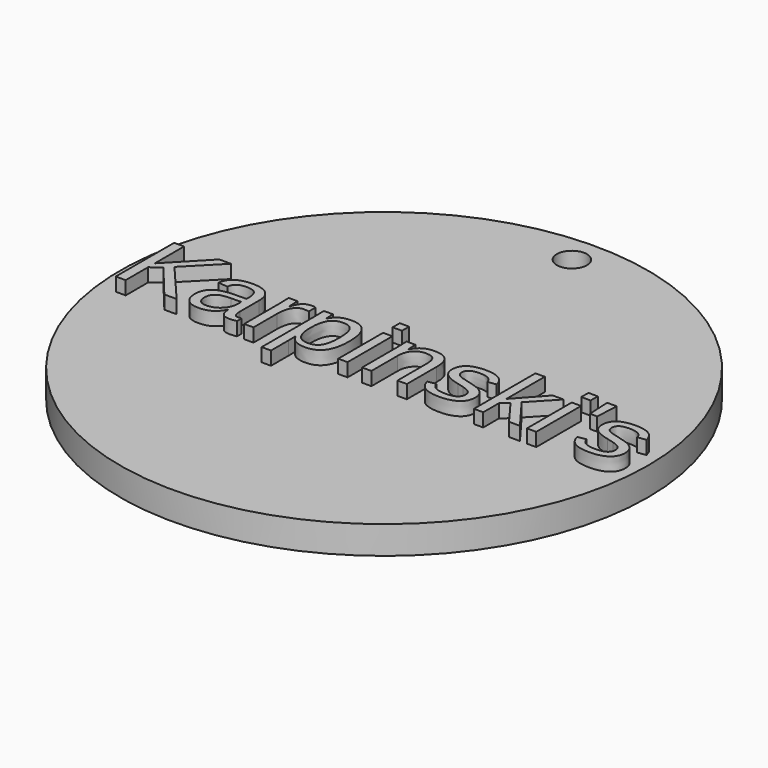
from build123d import *

# Parameters (mm, degrees)
F0_R         = 59.8348431243
F1_DEPTH     = 6.35
F2_TEXT_SIZE = 24.0505336827
F3_DEPTH     = 3.048
F4_R         = 3.4124645747
F5_DEPTH     = 25.4


# Not quite as in the source:
# - Text() gives the source's letters only with a copy of the font that has no kerning and outlines rounded to 1/6400 em; it was checked with that copy


with BuildPart() as f1:
    # F0 (on Top) → F1 (new body)
    with BuildSketch(Plane.XY):
        Circle(F0_R)
    extrude(amount=F1_DEPTH)

    # F2 (on face) → F3 (join)
    with BuildSketch(Plane.XY.offset(6.35)):
        with Locations((-57.3304596662, -6.8359926914)):
            Text("Karpinski's", F2_TEXT_SIZE, font='Arimo', text_align=(TextAlign.LEFT, TextAlign.BOTTOM))
    extrude(amount=F3_DEPTH)

    # F4 (on face) → F5 (cut)
    with BuildSketch(Plane.XY.offset(6.35)):
        with Locations((0, 53.221732378)):
            Circle(F4_R)
    extrude(amount=-F5_DEPTH, mode=Mode.SUBTRACT)


solid = f1.part
